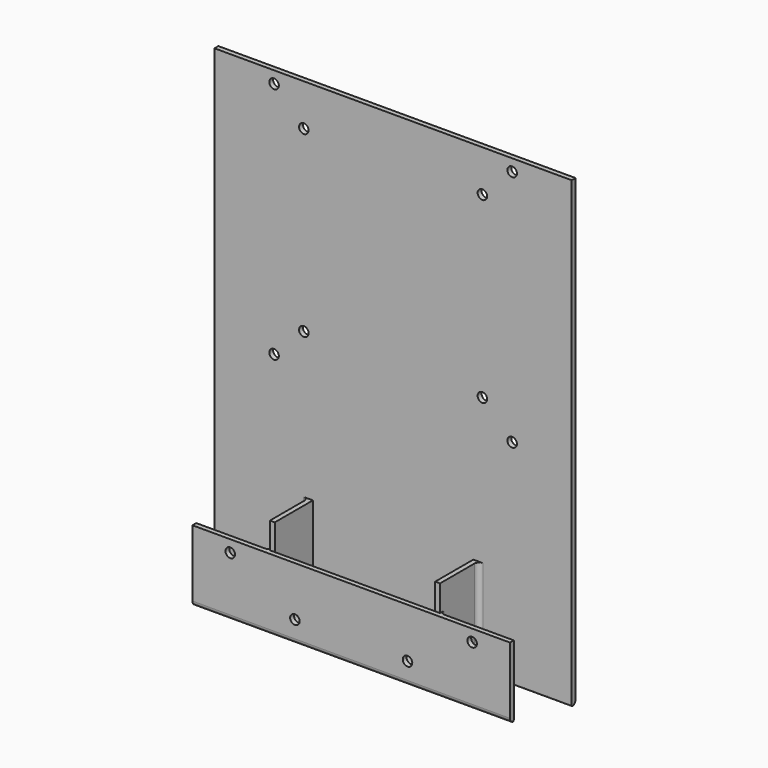
from build123d import *

# Parameters (mm, degrees)
F0_W     = 150
F0_H     = 194.7
F0_R     = 2
F1_DEPTH = 2.032
F2_W     = 20
F2_H     = 2
F3_DEPTH = 35.71875
F4_DEPTH = 66.675
F5_R     = 2
F6_DEPTH = 2
F7_W     = 2.032
F7_H     = 20
F8_DEPTH = 39
F9_R     = 2
F10_R    = 1.99999
F11_R    = 0.5


# Not quite as in the source:
# - a fillet or chamfer is up to 0.001 mm smaller than in the source, because OpenCascade refuses the exact size


with BuildPart() as f1:
    # F0 (on Front) → F1 (new body)
    with BuildSketch(Plane.XZ):
        with Locations((0, -42.35)):
            Rectangle(F0_W, F0_H)
        with Locations((-50, -50)):
            Circle(F0_R, mode=Mode.SUBTRACT)
        with Locations((50, -50)):
            Circle(F0_R, mode=Mode.SUBTRACT)
        with Locations((-37.5, -37.5)):
            Circle(F0_R, mode=Mode.SUBTRACT)
        with Locations((-50, 50)):
            Circle(F0_R, mode=Mode.SUBTRACT)
        with Locations((-37.5, 37.5)):
            Circle(F0_R, mode=Mode.SUBTRACT)
        with Locations((37.5, -37.5)):
            Circle(F0_R, mode=Mode.SUBTRACT)
        with Locations((37.5, 37.5)):
            Circle(F0_R, mode=Mode.SUBTRACT)
        with Locations((50, 50)):
            Circle(F0_R, mode=Mode.SUBTRACT)
    extrude(amount=F1_DEPTH)

    # F2 (on Right) → F3 (join, symmetric)
    with BuildSketch(Plane.YZ):
        with Locations((-12.032, -138.7)):
            Rectangle(F2_W, F2_H)
    extrude(amount=F3_DEPTH, both=True)

    # F2 (on Right) → F4 (join, symmetric)
    with BuildSketch(Plane.YZ):
        Polygon((-24.032, -139.7), (-22.032, -139.7), (-22.032, -137.7), (-22.032, -109.7), (-24.032, -109.7), align=None)
    extrude(amount=F4_DEPTH, both=True)

    # F5 (on face) → F6 (cut, through all)
    with BuildSketch(Plane.XZ.offset(24.032)):
        with Locations((-50.8, -114.7)):
            Circle(F5_R)
        with Locations((-23.6466728747, -130.575)):
            Circle(F5_R)
        with Locations((50.8, -114.7)):
            Circle(F5_R)
        with Locations((23.6466728747, -130.575)):
            Circle(F5_R)
    extrude(amount=-F6_DEPTH, mode=Mode.SUBTRACT)

    # F7 (on face) → F8 (join)
    with BuildSketch(Plane.XY.offset(-137.7)):
        with Locations((-34.70275, -12.032)):
            Rectangle(F7_W, F7_H)
        with Locations((34.70275, -12.032)):
            Rectangle(F7_W, F7_H)
    extrude(amount=F8_DEPTH)

    # F9
    f9_edges = [f1.edges().sort_by_distance(p)[0] for p in [
        (35.71875, -2.032, -119.2),
        (35.71875, -22.032, -124.7),
        (-35.71875, -2.032, -119.2),
        (-35.71875, -22.032, -124.7),
    ]]
    fillet(f9_edges, radius=F9_R)

    # F10 (radius 2 in the source; OpenCascade refuses exactly that, so slightly less here)
    f10_edges = [f1.edges().sort_by_distance(p)[0] for p in [
        (0, 0, -139.7),
        (0, -24.032, -139.7),
    ]]
    fillet(f10_edges, radius=F10_R)

    # F11
    f11_edges = [f1.edges().sort_by_distance(p)[0] for p in [
        (-35.71875, -12.032, -139.7),
        (35.71875, -12.032, -139.7),
        (33.68675, -12.032, -137.7),
        (-33.68675, -12.032, -137.7),
    ]]
    fillet(f11_edges, radius=F11_R)


solid = f1.part
